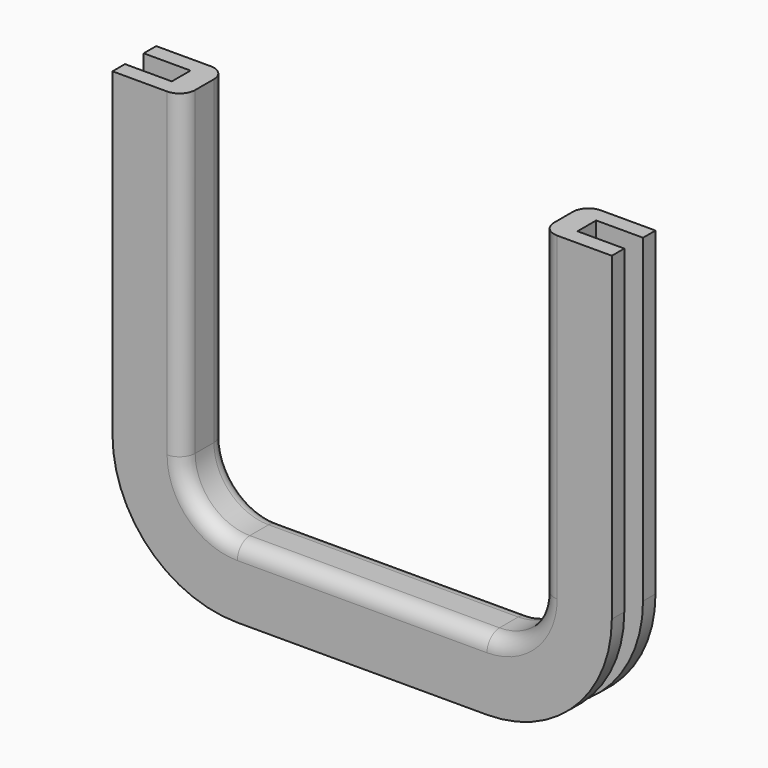
from build123d import *

# Parameters (mm, degrees)
F1_DEPTH = 1.5
F3_DEPTH = 1
F5_DEPTH = 1
F6_R     = 0.99999


# Not quite as in the source:
# - a fillet or chamfer is up to 0.001 mm smaller than in the source, because OpenCascade refuses the exact size
# - ends of sketch curves that miss each other by under 0.0002 mm in the source are joined


with BuildPart() as f1:
    # F0 (on Front) → F1 (new body)
    with BuildSketch(Plane.XZ):
        with BuildLine():
            Line((1.5, 25.5), (0, 25.5))
            Line((0, 25.5), (0, 5))
            ThreePointArc((0, 5), (1.4644660941, 1.4644660941), (5, 0))
            Line((5, 0), (21, 0))
            ThreePointArc((21, 0), (24.5355339059, 1.4644660941), (26, 5))
            Line((26, 5), (26, 25.5))
            Line((26, 25.5), (24.5, 25.5))
            Line((24.5, 25.5), (24.5, 5))
            ThreePointArc((24.5, 5), (23.4748737342, 2.5251262658), (21, 1.5))
            Line((21, 1.5), (5, 1.5))
            ThreePointArc((5, 1.5), (2.5251262658, 2.5251262658), (1.5, 5))
            Line((1.5, 5), (1.5, 25.5))
        make_face()
    extrude(amount=F1_DEPTH)

    # F2 (on face) → F3 (join)
    with BuildSketch(Plane.XZ.offset(1.5)):
        with BuildLine():
            Line((1.5, 5), (1.5, 25.5))
            Line((1.5, 25.5), (-3, 25.5))
            Line((-3, 25.5), (-3, 4.9999991806))
            ThreePointArc((-3, 4.9999991806), (-0.6568544895, -0.6568544895), (4.9999991806, -3))
            Line((4.9999991806, -3), (21, -3))
            ThreePointArc((21, -3), (26.6568542495, -0.6568542495), (29, 5))
            Line((29, 5), (29, 25.5))
            Line((29, 25.5), (24.5, 25.5))
            Line((24.5, 25.5), (24.5, 5))
            ThreePointArc((24.5, 5), (23.4748737342, 2.5251262658), (21, 1.5))
            Line((21, 1.5), (5, 1.5))
            ThreePointArc((5, 1.5), (2.5251257362, 2.5251263156), (1.5, 5))
        make_face()
    extrude(amount=F3_DEPTH)

    # F4 (on face) → F5 (join)
    with BuildSketch(Plane(origin=(0, 0, 0), x_dir=(-1, 0, 0), z_dir=(0, 1, 0))):
        with BuildLine():
            Line((-24.5, 5), (-24.5, 25.5))
            Line((-24.5, 25.5), (-29, 25.5))
            Line((-29, 25.5), (-29, 5))
            ThreePointArc((-29, 5), (-26.6568542495, -0.6568542495), (-21, -3))
            Line((-21, -3), (-5, -3))
            ThreePointArc((-5, -3), (0.6568542495, -0.6568542495), (3, 5))
            Line((3, 5), (3, 25.5))
            Line((3, 25.5), (-1.5, 25.5))
            Line((-1.5, 25.5), (-1.5, 5))
            ThreePointArc((-1.5, 5), (-2.5251262658, 2.5251262658), (-5, 1.5))
            Line((-5, 1.5), (-21, 1.5))
            ThreePointArc((-21, 1.5), (-23.4748737342, 2.5251262658), (-24.5, 5))
        make_face()
    extrude(amount=F5_DEPTH)

    # F6 (radius 1 in the source; OpenCascade refuses exactly that, so slightly less here)
    f6_edges = [f1.edges().sort_by_distance(p)[0] for p in [
        (23.474874, 1, 2.525126),
        (24.5, -2.5, 15.25),
    ]]
    fillet(f6_edges, radius=F6_R)


solid = f1.part
